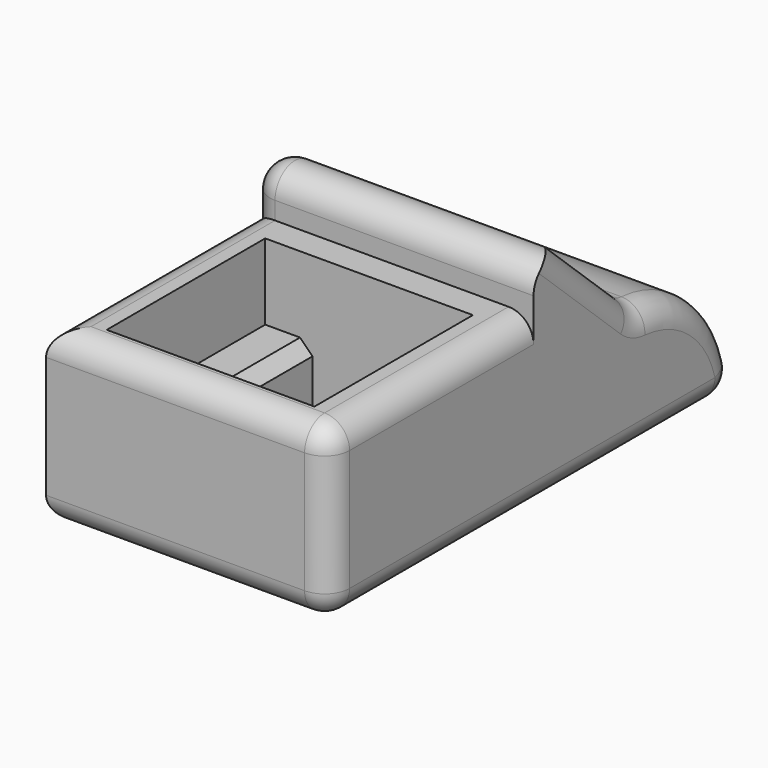
from build123d import *

# Parameters (mm, degrees)
F0_W     = 57.6730370522
F0_H     = 103.7285923958
F1_DEPTH = 50.1204133034
F2_W     = 51.8642961979
F2_H     = 15.2675881982
F3_DEPTH = 280.9666395187
F4_W     = 42.251765728
F4_H     = 40.2974346653
F5_DEPTH = 28.219755739
F6_W     = 9.6290325746
F6_H     = 40.2974346653
F7_DEPTH = 12.7694699913
F8_W     = 9.6542518586
F8_H     = 40.2974346653
F9_DEPTH = 10.5208531022
F10_R    = 5.08
F11_SIZE = 2.54


with BuildPart() as f1:
    # F0 (on Top) → F1 (new body)
    with BuildSketch(Plane.XY):
        Rectangle(F0_W, F0_H)
    extrude(amount=F1_DEPTH)

    # F2 (on face) → F3 (cut)
    with BuildSketch(Plane.YZ.offset(28.8365185261)):
        with BuildLine():
            ThreePointArc((26.9694030285, 25.0602066517), (44.5827153367, 17.6618916268), (51.8642961979, 0))
            Line((51.8642961979, 0), (51.8642961979, 50.1204133034))
            Line((51.8642961979, 50.1204133034), (0, 50.1204133034))
            Line((0, 50.1204133034), (26.9694030285, 25.0602066517))
        make_face()
        with Locations((-25.9321480989, 42.4866192043)):
            Rectangle(F2_W, F2_H)
    extrude(amount=-F3_DEPTH, mode=Mode.SUBTRACT)

    # F4 (on face) → F5 (cut)
    with BuildSketch(Plane.XY.offset(34.8528251052)):
        with Locations((0, -25.9321480989)):
            Rectangle(F4_W, F4_H)
    extrude(amount=-F5_DEPTH, mode=Mode.SUBTRACT)

    # F6 (on face) → F7 (join)
    with BuildSketch(Plane.XY.offset(6.6330693662)):
        with Locations((-16.3113665767, -25.9321480989)):
            Rectangle(F6_W, F6_H)
    extrude(amount=F7_DEPTH)

    # F8 (on face) → F9 (join)
    with BuildSketch(Plane.XY.offset(6.6330693662)):
        with Locations((16.2987569347, -25.9321480989)):
            Rectangle(F8_W, F8_H)
    extrude(amount=F9_DEPTH)

    # F10
    f10_edges = [f1.edges().sort_by_distance(p)[0] for p in [
        (28.836519, 44.582715, 17.661892),
        (28.836519, 13.484702, 37.59031),
        (0, 26.969403, 25.060207),
        (-28.836519, 13.484702, 37.59031),
        (-28.836519, 44.582715, 17.661892),
        (0, 51.864296, 0),
        (28.836519, 0, 0),
        (28.836519, -25.932148, 34.852825),
        (28.836519, -51.864296, 17.426413),
        (-28.836519, -25.932148, 34.852825),
        (0, -51.864296, 34.852825),
        (0, -51.864296, 0),
        (-28.836519, 0, 0),
        (-28.836519, 0, 42.486619),
        (0, 0, 50.120413),
    ]]
    fillet(f10_edges, radius=F10_R)

    # F11
    f11_edges = [f1.edges().sort_by_distance(p)[0] for p in [
        (-11.49685, -25.932148, 19.402539),
        (11.471631, -25.932148, 17.153922),
    ]]
    chamfer(f11_edges, length=F11_SIZE)


solid = f1.part
